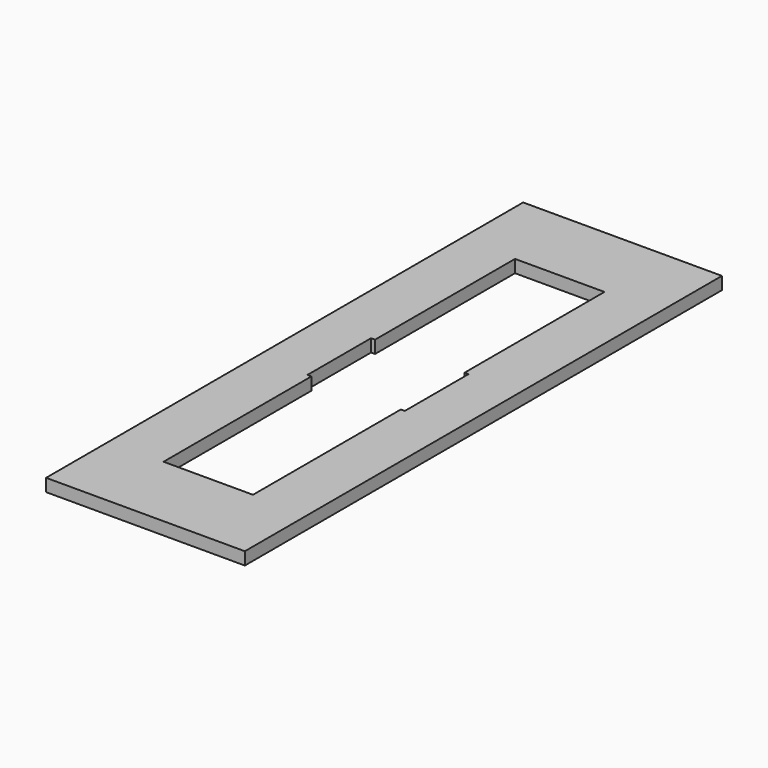
from build123d import *

# Parameters (mm, degrees)
F0_W     = 100
F0_H     = 300
F1_DEPTH = 6.35
F2_W     = 2
F2_H     = 40
F3_DEPTH = 25.4


# Not quite as in the source:
# - a length typed as a fraction of an inch, garbled in the dataset ("3 / 203.2 mm" for 3/8 in), is restored


with BuildPart() as f1:
    # F0 (on Top) → F1 (new body)
    with BuildSketch(Plane.XY):
        Rectangle(F0_W, F0_H)
    extrude(amount=F1_DEPTH)

    # F2 (on face) → F3 (cut)
    with BuildSketch(Plane.XY.offset(6.35)):
        Polygon((22.5, 22.48), (22.5, 110.5), (-22.5, 110.5), (-22.5, 22.48), (-22.5, -17.52), (-22.5, -110.5), (22.5, -110.5), (22.5, -17.52), align=None)
        with Locations((23.5, 2.48)):
            Rectangle(F2_W, F2_H)
        with Locations((-23.5, 2.48)):
            Rectangle(F2_W, F2_H)
    extrude(amount=-F3_DEPTH, mode=Mode.SUBTRACT)


solid = f1.part
